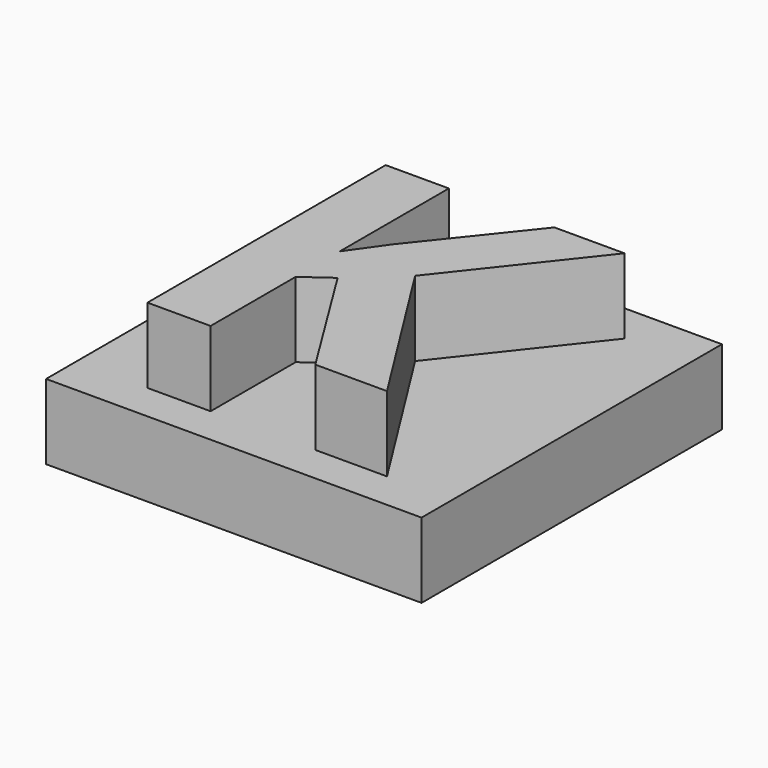
from build123d import *

# Parameters (mm, degrees)
F0_W         = 10
F0_H         = 10
F1_DEPTH     = 2
F2_TEXT_SIZE = 11.1111111111
F3_DEPTH     = 2


# Not quite as in the source:
# - Text() gives the source's letters only with a copy of the font that has no kerning and outlines rounded to 1/6400 em; it was checked with that copy


with BuildPart() as f1:
    # F0 (on Top) → F1 (new body)
    with BuildSketch(Plane.XY):
        Rectangle(F0_W, F0_H)
    extrude(amount=F1_DEPTH)

    # F2 (on face) → F3 (join)
    with BuildSketch(Plane.XY.offset(2)):
        with Locations((-4.0989583333, -4)):
            Text('K', F2_TEXT_SIZE, font='Open Sans', font_style=FontStyle.BOLD, text_align=(TextAlign.LEFT, TextAlign.BOTTOM))
    extrude(amount=F3_DEPTH)


solid = f1.part
